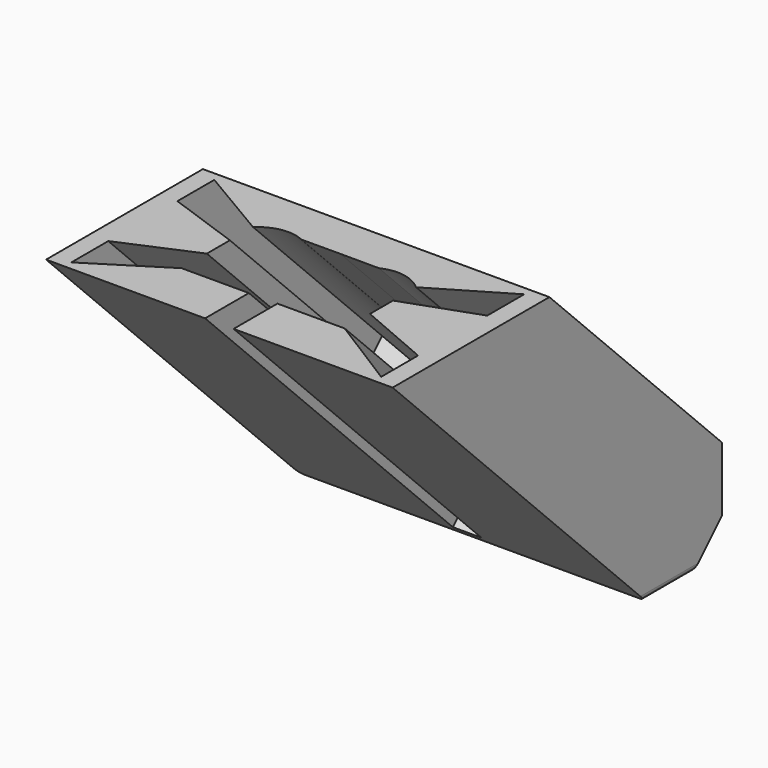
from build123d import *

# Parameters (mm, degrees)
F0_W     = 43.18
F0_H     = 17.272
F2_DEPTH = 76.2
F3_DEPTH = 69.85
F6_ANGLE = 45
F8_W     = 97.1712954342
F8_H     = 80.9760764241
F8_W_2   = 68.9119933241
F8_H_2   = 39.37
F9_DEPTH = 38.1
F10_R    = 0.762


# Not quite as in the source:
# - ends of sketch curves that miss each other by under 0.0002 mm in the source are joined


with BuildPart() as f2:
    # F0 (on Front) → F2 (new body)
    with BuildSketch(Plane.XZ):
        Rectangle(F0_W, F0_H)
    extrude(amount=-F2_DEPTH)

    # F1 (on Front) → F3 (cut)
    with BuildSketch(Plane.XZ):
        with BuildLine():
            Line((10.1640512741, -1.0311319662), (10.1640512741, 1.5088680338))
            Line((10.1640512741, 1.5088680338), (19.304, 3.81))
            Line((19.304, 3.81), (19.304, 7.874))
            Line((19.304, 7.874), (10.1640512741, 4.0488680338))
            ThreePointArc((10.1640512741, 4.0488680338), (7.567989059, 4.950925683), (4.8339106143, 4.6715297537))
            Line((4.8339106143, 4.6715297537), (1.97346e-05, 4.6852644338))
            Line((1.97346e-05, 4.6852644338), (-4.8339106143, 4.6715297537))
            ThreePointArc((-4.8339106143, 4.6715297537), (-7.567989059, 4.950925683), (-10.1640512741, 4.0488680338))
            Line((-10.1640512741, 4.0488680338), (-19.304, 7.874))
            Line((-19.304, 7.874), (-19.304, 3.81))
            Line((-19.304, 3.81), (-10.1640512741, 1.5088680338))
            Line((-10.1640512741, 1.5088680338), (-10.1640512741, -1.0311319662))
            Line((-10.1640512741, -1.0311319662), (-19.304, -3.81))
            Line((-19.304, -3.81), (-19.304, -7.874))
            Line((-19.304, -7.874), (-10.1640512741, -3.81))
            Line((-10.1640512741, -3.81), (-1.778, -3.81))
            Line((-1.778, -3.81), (-1.778, -7.874))
            Line((-1.778, -7.874), (-1.778, -8.9796995744))
            Line((-1.778, -8.9796995744), (1.778, -8.9796995744))
            Line((1.778, -8.9796995744), (1.778, -7.874))
            Line((1.778, -7.874), (1.778, -3.81))
            Line((1.778, -3.81), (10.1640512741, -3.81))
            Line((10.1640512741, -3.81), (19.304, -7.874))
            Line((19.304, -7.874), (19.304, -3.81))
            Line((19.304, -3.81), (10.1640512741, -1.0311319662))
        make_face()
    extrude(amount=-F3_DEPTH, mode=Mode.SUBTRACT)


with BuildPart() as f2_1:
    # F4: moved
    add(f2.part.moved(Location((0, -38.1, 0))))


with BuildPart() as f2_2:
    # F6: moved
    add(f2_1.part.rotate(Axis((-4.1610468179, 0, 0), (-1, 0, 0)), F6_ANGLE))

    # F8 (on Right) → F9 (cut, symmetric)
    with BuildSketch(Plane.YZ):
        with Locations((-6.1953347176, -4.1167326272)):
            Rectangle(F8_W, F8_H)
        with Locations((-5.4169551435, -9.6378130603)):
            Rectangle(F8_W_2, F8_H_2, mode=Mode.SUBTRACT)
    extrude(amount=F9_DEPTH, both=True, mode=Mode.SUBTRACT)

    # F10
    f10_edges = [f2_2.edges().sort_by_distance(p)[0] for p in [
        (21.59, 20.834194, -29.322813),
        (-21.59, 20.834194, -29.322813),
    ]]
    fillet(f10_edges, radius=F10_R)


solid = f2_2.part
